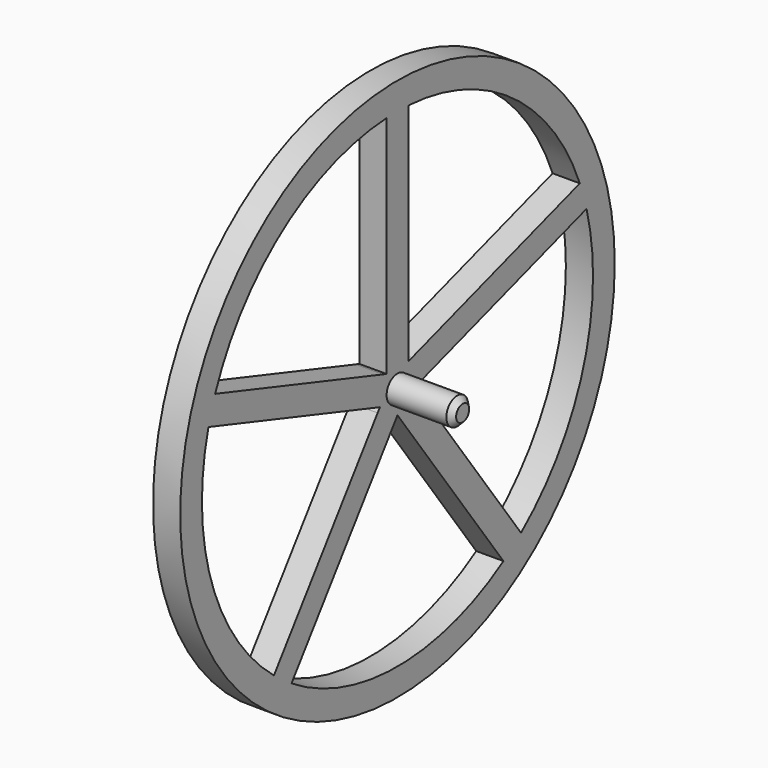
from build123d import *

# Parameters (mm, degrees)
F0_R     = 50
F1_DEPTH = 2.5
F2_R     = 2.5
F3_DEPTH = 12
F4_SIZE  = 1


with BuildPart() as f1:
    # F0 (on Right) → F1 (new body, symmetric)
    with BuildSketch(Plane.YZ):
        Circle(F0_R)
        with BuildLine():
            ThreePointArc((2.5, 44.930501889), (26.4503363532, 36.4057647469), (41.958904116, 16.2619299402))
            ThreePointArc((41.958904116, 16.2619299402), (42.7975432333, 13.9057647469), (43.5039890879, 11.5066473588))
            ThreePointArc((43.5039890879, 11.5066473588), (44.6244300185, 5.8017450411), (45, 0))
            ThreePointArc((45, 0), (40.6475171403, -19.3074946672), (28.4320288744, -34.8800764633))
            ThreePointArc((28.4320288744, -34.8800764633), (26.4503363532, -36.4057647469), (24.3869439025, -37.8190027248))
            ThreePointArc((24.3869439025, -37.8190027248), (0, -45), (-24.3869439025, -37.8190027248))
            ThreePointArc((-24.3869439025, -37.8190027248), (-26.4503363532, -36.4057647469), (-28.4320288744, -34.8800764633))
            ThreePointArc((-28.4320288744, -34.8800764633), (-42.7975432333, -13.9057647469), (-43.5039890879, 11.5066473588))
            ThreePointArc((-43.5039890879, 11.5066473588), (-42.7975432333, 13.9057647469), (-41.958904116, 16.2619299402))
            ThreePointArc((-41.958904116, 16.2619299402), (-26.4503363532, 36.4057647469), (-2.5, 44.930501889))
            ThreePointArc((-2.5, 44.930501889), (0, 45), (2.5, 44.930501889))
        make_face(mode=Mode.SUBTRACT)
        with BuildLine():
            ThreePointArc((-2.5, 4.3301270189), (0, 5), (2.5, 4.3301270189))
            Line((2.5, 4.3301270189), (2.5, 44.930501889))
            ThreePointArc((2.5, 44.930501889), (0, 45), (-2.5, 44.930501889))
            Line((-2.5, 44.930501889), (-2.5, 4.3301270189))
        make_face()
        with BuildLine():
            ThreePointArc((-4.8907380037, -1.0395584541), (-4.7552825815, 1.5450849719), (-3.3456530318, 3.7157241274))
            Line((-3.3456530318, 3.7157241274), (-41.958904116, 16.2619299402))
            ThreePointArc((-41.958904116, 16.2619299402), (-42.7975432333, 13.9057647469), (-43.5039890879, 11.5066473588))
            Line((-43.5039890879, 11.5066473588), (-4.8907380037, -1.0395584541))
        make_face()
        with BuildLine():
            Line((-24.3869439025, -37.8190027248), (-0.5226423163, -4.9726094768))
            ThreePointArc((-0.5226423163, -4.9726094768), (-2.9389262615, -4.0450849719), (-4.5677272882, -2.0336832154))
            Line((-4.5677272882, -2.0336832154), (-28.4320288744, -34.8800764633))
            ThreePointArc((-28.4320288744, -34.8800764633), (-26.4503363532, -36.4057647469), (-24.3869439025, -37.8190027248))
        make_face()
        with BuildLine():
            Line((28.4320288744, -34.8800764633), (4.5677272882, -2.0336832154))
            ThreePointArc((4.5677272882, -2.0336832154), (2.9389262615, -4.0450849719), (0.5226423163, -4.9726094768))
            Line((0.5226423163, -4.9726094768), (24.3869439025, -37.8190027248))
            ThreePointArc((24.3869439025, -37.8190027248), (26.4503363532, -36.4057647469), (28.4320288744, -34.8800764633))
        make_face()
        with BuildLine():
            ThreePointArc((3.3456530318, 3.7157241274), (4.5677272882, 2.0336832154), (5, 0))
            ThreePointArc((5, 0), (4.9726094768, -0.5226423163), (4.8907380037, -1.0395584541))
            Line((4.8907380037, -1.0395584541), (43.5039890879, 11.5066473588))
            ThreePointArc((43.5039890879, 11.5066473588), (42.7975432333, 13.9057647469), (41.958904116, 16.2619299402))
            Line((41.958904116, 16.2619299402), (3.3456530318, 3.7157241274))
        make_face()
        Polygon((2.5, 0.8122992406), (2.5, 3.4409548012), (0, 2.6286555606), (-2.5, 3.4409548012), (-2.5, 0.8122992406), (-4.0450849719, -1.3143277803), (-1.5450849719, -2.1266270209), (0, -4.2532540418), (1.5450849719, -2.1266270209), (4.0450849719, -1.3143277803), align=None)
        with BuildLine():
            Line((2.5, 3.4409548012), (2.5, 4.3301270189))
            ThreePointArc((2.5, 4.3301270189), (0, 5), (-2.5, 4.3301270189))
            Line((-2.5, 4.3301270189), (-2.5, 3.4409548012))
            Line((-2.5, 3.4409548012), (0, 2.6286555606))
            Line((0, 2.6286555606), (2.5, 3.4409548012))
        make_face()
        with BuildLine():
            Line((-2.5, 3.4409548012), (-3.3456530318, 3.7157241274))
            ThreePointArc((-3.3456530318, 3.7157241274), (-4.7552825815, 1.5450849719), (-4.8907380037, -1.0395584541))
            Line((-4.8907380037, -1.0395584541), (-4.0450849719, -1.3143277803))
            Line((-4.0450849719, -1.3143277803), (-2.5, 0.8122992406))
            Line((-2.5, 0.8122992406), (-2.5, 3.4409548012))
        make_face()
        with BuildLine():
            ThreePointArc((-4.5677272882, -2.0336832154), (-2.9389262615, -4.0450849719), (-0.5226423163, -4.9726094768))
            Line((-0.5226423163, -4.9726094768), (0, -4.2532540418))
            Line((0, -4.2532540418), (-1.5450849719, -2.1266270209))
            Line((-1.5450849719, -2.1266270209), (-4.0450849719, -1.3143277803))
            Line((-4.0450849719, -1.3143277803), (-4.5677272882, -2.0336832154))
        make_face()
        with BuildLine():
            ThreePointArc((0.5226423163, -4.9726094768), (2.9389262615, -4.0450849719), (4.5677272882, -2.0336832154))
            Line((4.5677272882, -2.0336832154), (4.0450849719, -1.3143277803))
            Line((4.0450849719, -1.3143277803), (1.5450849719, -2.1266270209))
            Line((1.5450849719, -2.1266270209), (0, -4.2532540418))
            Line((0, -4.2532540418), (0.5226423163, -4.9726094768))
        make_face()
        with BuildLine():
            ThreePointArc((4.8907380037, -1.0395584541), (4.9726094768, -0.5226423163), (5, 0))
            ThreePointArc((5, 0), (4.5677272882, 2.0336832154), (3.3456530318, 3.7157241274))
            Line((3.3456530318, 3.7157241274), (2.5, 3.4409548012))
            Line((2.5, 3.4409548012), (2.5, 0.8122992406))
            Line((2.5, 0.8122992406), (4.0450849719, -1.3143277803))
            Line((4.0450849719, -1.3143277803), (4.8907380037, -1.0395584541))
        make_face()
    extrude(amount=F1_DEPTH, both=True)

    # F2 (on face) → F3 (join)
    with BuildSketch(Plane.YZ.offset(2.5)):
        Circle(F2_R)
    extrude(amount=F3_DEPTH)

    # F4
    f4_edges = [f1.edges().sort_by_distance(p)[0] for p in [
        (14.5, -2.5, 0),
    ]]
    chamfer(f4_edges, length=F4_SIZE)


solid = f1.part
